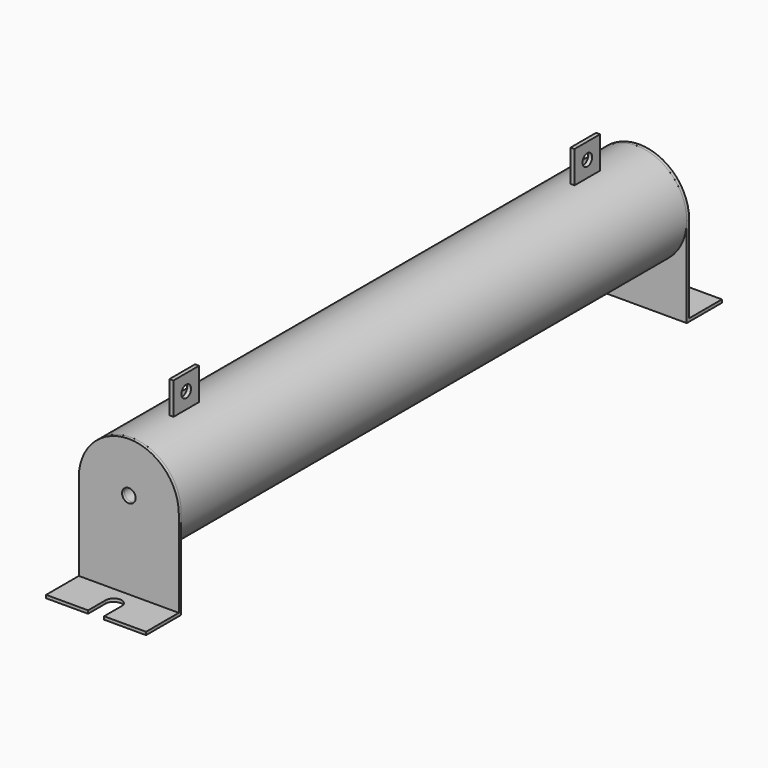
from build123d import *

# Parameters (mm, degrees)
F0_R      = 25
F1_DEPTH  = 316
F3_DEPTH  = 1.524
F4_W      = 50
F4_H      = 22
F5_DEPTH  = 1.524
F7_DEPTH  = 1.524
F9_DEPTH  = 1.524
F10_W     = 50
F10_H     = 20.476
F11_DEPTH = 1.524
F13_DEPTH = 1.524
F14_W     = 16
F14_H     = 16
F15_DEPTH = 2
F17_D     = 6
F18_W     = 16
F18_H     = 16
F19_DEPTH = 2
F21_D     = 6
F23_D     = 6.7564
F23_2_D   = 6.7564
F23_3_D   = 6.7564


# Not quite as in the source:
# - a pattern or mirror of a feature is missing from the dataset's text; its kind, count and spacing are read off the source's solid


with BuildPart() as f1:
    # F0 (on Front) → F1 (new body)
    with BuildSketch(Plane.XZ):
        Circle(F0_R)
    extrude(amount=-F1_DEPTH)

    # F23 (through all)
    with Locations(Plane.XZ.offset(1.524)):
        with Locations((0, 0)):
            Hole(F23_D / 2)


with BuildPart() as f3:
    # F2 (on Front) → F3 (new body)
    with BuildSketch(Plane.XZ):
        with BuildLine():
            Line((-25, 0), (25, 0))
            ThreePointArc((25, 0), (0, 25), (-25, 0))
        make_face()
        with BuildLine():
            Line((25, -45), (25, 0))
            ThreePointArc((25, 0), (0, -25), (-25, 0))
            Line((-25, 0), (-25, -45))
            Line((-25, -45), (25, -45))
        make_face()
        with BuildLine():
            ThreePointArc((-25, 0), (0, -25), (25, 0))
            Line((25, 0), (-25, 0))
        make_face()
    extrude(amount=F3_DEPTH)

    # F4 (on face) → F5 (join)
    with BuildSketch(Plane(origin=(0, 0, -45), x_dir=(1, 0, 0), z_dir=(0, 0, -1))):
        with Locations((0, 11)):
            Rectangle(F4_W, F4_H)
    extrude(amount=-F5_DEPTH)

    # F6 (on face) → F7 (cut)
    with BuildSketch(Plane(origin=(0, 0, -45), x_dir=(1, 0, 0), z_dir=(0, 0, -1))):
        with BuildLine():
            Line((-4, 11), (4, 11))
            ThreePointArc((4, 11), (0, 15), (-4, 11))
        make_face()
        with BuildLine():
            ThreePointArc((-4, 11), (0, 7), (4, 11))
            Line((4, 11), (-4, 11))
        make_face()
        with BuildLine():
            ThreePointArc((-4, 11), (0, 15), (4, 11))
            Line((4, 11), (4, 22))
            Line((4, 22), (-4, 22))
            Line((-4, 22), (-4, 11))
        make_face()
    extrude(amount=-F7_DEPTH, mode=Mode.SUBTRACT)

    # F23#2 (through all)
    with Locations(Plane.XZ.offset(1.524)):
        with Locations((0, 0)):
            Hole(F23_2_D / 2)


with BuildPart() as f9:
    # F8 (on face) → F9 (new body)
    with BuildSketch(Plane(origin=(0, 316, 0), x_dir=(-1, 0, 0), z_dir=(0, 1, 0))):
        with BuildLine():
            Line((-25, 0), (25, 0))
            ThreePointArc((25, 0), (0, 25), (-25, 0))
        make_face()
        with BuildLine():
            Line((25, -45), (25, 0))
            ThreePointArc((25, 0), (0, -25), (-25, 0))
            Line((-25, 0), (-25, -45))
            Line((-25, -45), (25, -45))
        make_face()
        with BuildLine():
            ThreePointArc((-25, 0), (0, -25), (25, 0))
            Line((25, 0), (-25, 0))
        make_face()
    extrude(amount=F9_DEPTH)

    # F10 (on face) → F11 (join)
    with BuildSketch(Plane(origin=(0, 0, -45), x_dir=(1, 0, 0), z_dir=(0, 0, -1))):
        with Locations((0, -327.762)):
            Rectangle(F10_W, F10_H)
    extrude(amount=-F11_DEPTH)

    # F12 (on face) → F13 (cut)
    with BuildSketch(Plane(origin=(0, 0, -45), x_dir=(1, 0, 0), z_dir=(0, 0, -1))):
        with BuildLine():
            Line((-4, -327), (4, -327))
            ThreePointArc((4, -327), (0, -323), (-4, -327))
        make_face()
        with BuildLine():
            Line((4, -338), (4, -327))
            ThreePointArc((4, -327), (0, -331), (-4, -327))
            Line((-4, -327), (-4, -338))
            Line((-4, -338), (4, -338))
        make_face()
        with BuildLine():
            ThreePointArc((-4, -327), (0, -331), (4, -327))
            Line((4, -327), (-4, -327))
        make_face()
    extrude(amount=-F13_DEPTH, mode=Mode.SUBTRACT)

    # F23#3 (through all)
    with Locations(Plane.XZ.offset(1.524)):
        with Locations((0, 0)):
            f23_3 = Hole(F23_3_D / 2)

    # F23_3_copies: F23#3 across plane
    add(f23_3.mirror(Plane.ZX.offset(158)), mode=Mode.SUBTRACT)


with BuildPart() as f15:
    # F14 (on Right) → F15 (new body)
    with BuildSketch(Plane.YZ):
        with Locations((31.876, 33)):
            Rectangle(F14_W, F14_H)
    extrude(amount=F15_DEPTH)

    # F17 (through all)
    with Locations(Plane.YZ.offset(2)):
        with Locations((31.876, 33)):
            Hole(F17_D / 2)


with BuildPart() as f19:
    # F18 (on Right) → F19 (new body)
    with BuildSketch(Plane.YZ):
        with Locations((282.6, 33)):
            Rectangle(F18_W, F18_H)
    extrude(amount=F19_DEPTH)

    # F21 (through all)
    with Locations(Plane(origin=(0, 0, 0), x_dir=(0, -1, 0), z_dir=(-1, 0, 0))):
        with Locations((-282.6, 33)):
            Hole(F21_D / 2)


solid = Compound([f1.part, f3.part, f9.part, f15.part, f19.part])
